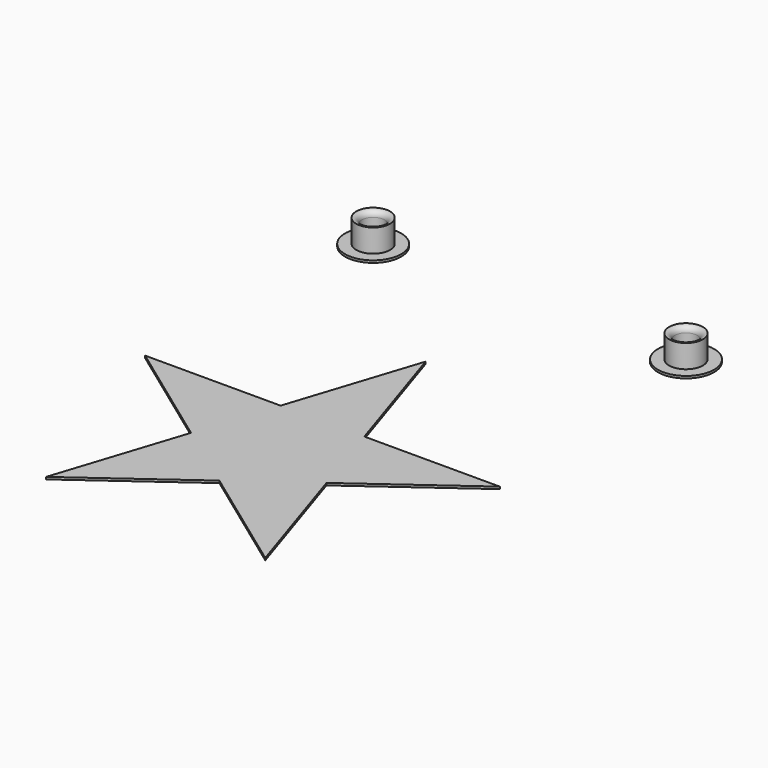
from build123d import *

# Parameters (mm, degrees)
F0_R     = 5
F0_R_2   = 3
F1_DEPTH = 0.4
F0_R_3   = 2
F2_DEPTH = 4.5
F3_R     = 0.99999
F3_2_R   = 0.99999
F5_DEPTH = 0.4


# Not quite as in the source:
# - a fillet or chamfer is up to 0.001 mm smaller than in the source, because OpenCascade refuses the exact size


with BuildPart() as f1:
    # F0 (on Top) → F1 (new body)
    with BuildSketch(Plane.XY):
        with Locations((-27.8231911361, 20.2907286584)):
            Circle(F0_R)
        with Locations((-27.8231911361, 20.2907286584)):
            Circle(F0_R_2, mode=Mode.SUBTRACT)
    extrude(amount=F1_DEPTH)

    # F0 (on Top) → F2 (join)
    with BuildSketch(Plane.XY):
        with Locations((-27.8231911361, 20.2907286584)):
            Circle(F0_R_2)
        with Locations((-27.8231911361, 20.2907286584)):
            Circle(F0_R_3, mode=Mode.SUBTRACT)
    extrude(amount=F2_DEPTH)

    # F3 (radius 1 in the source; OpenCascade refuses exactly that, so slightly less here)
    f3_edges = [f1.edges().sort_by_distance(p)[0] for p in [
        (-29.823191, 20.290729, 4.5),
        (-29.823191, 20.290729, 0),
    ]]
    fillet(f3_edges, radius=F3_R)


with BuildPart() as f1b:
    # F0 (on Top) → F1, piece 2 (new body)
    with BuildSketch(Plane.XY):
        with Locations((27.8231911361, 20.2907286584)):
            Circle(F0_R)
        with Locations((27.8231911361, 20.2907286584)):
            Circle(F0_R_2, mode=Mode.SUBTRACT)
    extrude(amount=F1_DEPTH)

    # F0 (on Top) → F2, piece 2 (join)
    with BuildSketch(Plane.XY):
        with Locations((27.8231911361, 20.2907286584)):
            Circle(F0_R_2)
        with Locations((27.8231911361, 20.2907286584)):
            Circle(F0_R_3, mode=Mode.SUBTRACT)
    extrude(amount=F2_DEPTH)

    # F3#2 (radius 1 in the source; OpenCascade refuses exactly that, so slightly less here)
    f3_2_edges = [f1b.edges().sort_by_distance(p)[0] for p in [
        (25.823191, 20.290729, 4.5),
        (25.823191, 20.290729, 0),
    ]]
    fillet(f3_2_edges, radius=F3_2_R)


with BuildPart() as f5:
    # F4 (on Top) → F5 (new body)
    with BuildSketch(Plane.XY):
        Polygon((-31.5438667271, -25.7632551613), (-12.0486849532, -39.9273338113), (-19.495181774, -62.8452944863), (0, -48.6812158363), (19.495181774, -62.8452944863), (12.0486849532, -39.9273338113), (31.5438667271, -25.7632551613), (7.4464968208, -25.7632551613), (0, -2.8452944863), (-7.4464968208, -25.7632551613), align=None)
    extrude(amount=F5_DEPTH)


solid = Compound([f1.part, f1b.part, f5.part])
